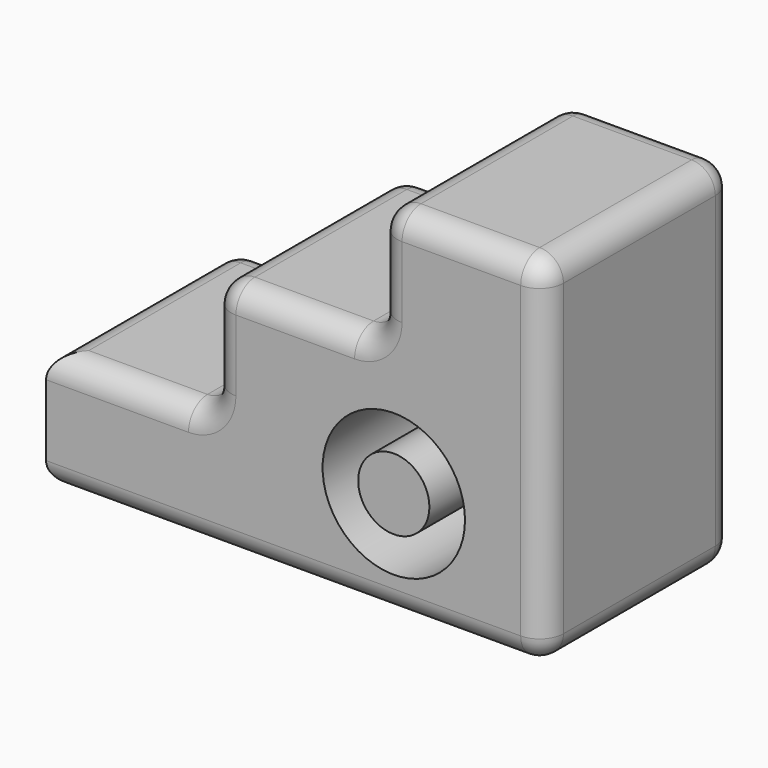
from build123d import *

# Parameters (mm, degrees)
F1_DEPTH      = 50
F2_R          = 15
F2_R_2        = 7.5
F3_DEPTH      = 50
F4_T3_DEPTH   = 50
F4_T6_DEPTH   = 50
F4_S9_W       = 5.1
F4_S9_H       = 5.1
F4_T10_DEPTH  = 5.1
F4_S14_W      = 5.1
F4_S14_H      = 5.1
F4_T15_DEPTH  = 5.1
F4_S19_W      = 5.1
F4_S19_H      = 5.1
F4_T20_DEPTH  = 5.1
F4_S24_W      = 5.1
F4_S24_H      = 5.1
F4_T25_DEPTH  = 5.1
F4_S29_W      = 5.1
F4_S29_H      = 5.1
F4_T30_DEPTH  = 5.1
F4_S34_W      = 5.1
F4_S34_H      = 5.1
F4_T35_DEPTH  = 5.1
F4_S39_W      = 5.1
F4_S39_H      = 5.1
F4_T40_DEPTH  = 5.1
F4_S44_W      = 5.1
F4_S44_H      = 5.1
F4_T45_DEPTH  = 5.1
F4_S49_W      = 5.1
F4_S49_H      = 5.1
F4_T50_DEPTH  = 5.1
F4_S54_W      = 5.1
F4_S54_H      = 5.1
F4_T55_DEPTH  = 5.1
F4_T60_DEPTH  = 57.5
F4_T63_DEPTH  = 40
F4_T66_DEPTH  = 40
F4_T69_DEPTH  = 40
F4_T72_DEPTH  = 25
F4_T75_DEPTH  = 25
F4_T78_DEPTH  = 25
F4_T81_DEPTH  = 42.5
F4_T84_DEPTH  = 25
F4_T87_DEPTH  = 25
F4_T93_DEPTH  = 112.5
F4_T96_DEPTH  = 57.5
F4_T99_DEPTH  = 40
F4_T102_DEPTH = 95
F4_T105_DEPTH = 65
F4_T108_DEPTH = 15
F4_T111_DEPTH = 65
F4_T114_DEPTH = 15
F4_T117_DEPTH = 15
F4_T120_DEPTH = 15
F4_T123_DEPTH = 15
F4_T126_ANGLE = 90
F4_T129_ANGLE = 90
F4_T132_ANGLE = 90
F4_T135_ANGLE = 90


# Not quite as in the source:
# - a fillet or chamfer that OpenCascade refuses, or shapes differently, is made with other operations: its cross-section is extruded or revolved along the edge and cut away or added


with BuildPart() as f1:
    # F0 (on Front) → F1 (new body)
    with BuildSketch(Plane.XZ):
        Polygon((-66.1900187428, 24.934796177), (-66.1900187428, -0.065203823), (38.8099812572, -0.065203823), (38.8099812572, 74.934796177), (3.8099812572, 74.934796177), (3.8099812572, 49.934796177), (-31.1900187428, 49.934796177), (-31.1900187428, 24.934796177), align=None)
    extrude(amount=F1_DEPTH)

    # F2 (on face) → F3 (cut, through all)
    with BuildSketch(Plane.XZ.offset(50)):
        with Locations((7.0711858571, 22.5817617029)):
            Circle(F2_R)
        with Locations((7.0711858571, 22.5817617029)):
            Circle(F2_R_2, mode=Mode.SUBTRACT)
    extrude(amount=-F3_DEPTH, mode=Mode.SUBTRACT)

    # F4: fillet of radius 5 on 24 edges, made by hand


with BuildPart() as f4_tool1:
    # F4_s2 → F4_t3 (new body)
    with BuildSketch(Plane.XZ):
        with BuildLine():
            ThreePointArc((-36.1900187428, 24.934796177), (-32.6544848368, 26.3992622711), (-31.1900187428, 29.934796177))
            Line((-31.1900187428, 29.934796177), (-31.1900187428, 24.934796177))
            Line((-31.1900187428, 24.934796177), (-36.1900187428, 24.934796177))
        make_face()
    extrude(amount=F4_T3_DEPTH)


with BuildPart() as f4_tool4:
    # F4_s5 → F4_t6 (new body)
    with BuildSketch(Plane.XZ):
        with BuildLine():
            ThreePointArc((3.8099812572, 54.934796177), (2.3455151632, 51.3992622711), (-1.1900187428, 49.934796177))
            Line((-1.1900187428, 49.934796177), (3.8099812572, 49.934796177))
            Line((3.8099812572, 49.934796177), (3.8099812572, 54.934796177))
        make_face()
    extrude(amount=F4_T6_DEPTH)


with BuildPart() as f1_1:
    add(f1.part)

    # F4_t7: union F4_tool1, F4_tool4
    add([f4_tool1.part, f4_tool4.part])


with BuildPart() as f4_tool8:
    # F4_s9 → F4_t10 (new body)
    with BuildSketch(Plane.YZ.offset(-61.1900187428)):
        with Locations((-2.45, 22.484796177)):
            Rectangle(F4_S9_W, F4_S9_H)
    extrude(amount=-F4_T10_DEPTH)

    # F4_s11 → F4_t12 (revolve, cut)
    with BuildSketch(Plane(origin=(-61.1900187428, -5, 19.934796177), x_dir=(0, -0.7071067812, -0.7071067812), z_dir=(0, 0.7071067812, -0.7071067812))):
        with BuildLine():
            ThreePointArc((0, -5), (5, 0), (0, 5))
            Line((0, 5), (0, -5))
        make_face()
    revolve(axis=Axis((-61.1900187428, -5, 19.934796177), (-1, 0, 0)), mode=Mode.SUBTRACT)


with BuildPart() as f4_tool13:
    # F4_s14 → F4_t15 (new body)
    with BuildSketch(Plane.XY.offset(44.934796177)):
        with Locations((-28.7400187428, -2.45)):
            Rectangle(F4_S14_W, F4_S14_H)
    extrude(amount=F4_T15_DEPTH)

    # F4_s16 → F4_t17 (revolve, cut)
    with BuildSketch(Plane(origin=(-26.1900187428, -5, 44.934796177), x_dir=(0.7071067812, -0.7071067812, 0), z_dir=(-0.7071067812, -0.7071067812, 0))):
        with BuildLine():
            ThreePointArc((0, -5), (5, 0), (0, 5))
            Line((0, 5), (0, -5))
        make_face()
    revolve(axis=Axis((-26.1900187428, -5, 44.934796177), (0, 0, 1)), mode=Mode.SUBTRACT)


with BuildPart() as f4_tool18:
    # F4_s19 → F4_t20 (new body)
    with BuildSketch(Plane.XY.offset(44.934796177)):
        with Locations((-28.7400187428, -47.55)):
            Rectangle(F4_S19_W, F4_S19_H)
    extrude(amount=F4_T20_DEPTH)

    # F4_s21 → F4_t22 (revolve, cut)
    with BuildSketch(Plane(origin=(-26.1900187428, -45, 44.934796177), x_dir=(0.7071067812, 0.7071067812, 0), z_dir=(0.7071067812, -0.7071067812, 0))):
        with BuildLine():
            ThreePointArc((0, -5), (5, 0), (0, 5))
            Line((0, 5), (0, -5))
        make_face()
    revolve(axis=Axis((-26.1900187428, -45, 44.934796177), (0, 0, 1)), mode=Mode.SUBTRACT)


with BuildPart() as f4_tool23:
    # F4_s24 → F4_t25 (new body)
    with BuildSketch(Plane.YZ.offset(8.8099812572)):
        with Locations((-2.45, 72.484796177)):
            Rectangle(F4_S24_W, F4_S24_H)
    extrude(amount=-F4_T25_DEPTH)

    # F4_s26 → F4_t27 (revolve, cut)
    with BuildSketch(Plane(origin=(8.8099812572, -5, 69.934796177), x_dir=(0, -0.7071067812, -0.7071067812), z_dir=(0, 0.7071067812, -0.7071067812))):
        with BuildLine():
            ThreePointArc((0, -5), (5, 0), (0, 5))
            Line((0, 5), (0, -5))
        make_face()
    revolve(axis=Axis((8.8099812572, -5, 69.934796177), (-1, 0, 0)), mode=Mode.SUBTRACT)


with BuildPart() as f4_tool28:
    # F4_s29 → F4_t30 (new body)
    with BuildSketch(Plane.YZ.offset(8.8099812572)):
        with Locations((-47.55, 72.484796177)):
            Rectangle(F4_S29_W, F4_S29_H)
    extrude(amount=-F4_T30_DEPTH)

    # F4_s31 → F4_t32 (revolve, cut)
    with BuildSketch(Plane(origin=(8.8099812572, -45, 69.934796177), x_dir=(0, 0.7071067812, -0.7071067812), z_dir=(0, 0.7071067812, 0.7071067812))):
        with BuildLine():
            ThreePointArc((0, -5), (5, 0), (0, 5))
            Line((0, 5), (0, -5))
        make_face()
    revolve(axis=Axis((8.8099812572, -45, 69.934796177), (-1, 0, 0)), mode=Mode.SUBTRACT)


with BuildPart() as f4_tool33:
    # F4_s34 → F4_t35 (new body)
    with BuildSketch(Plane.YZ.offset(33.8099812572)):
        with Locations((-2.45, 72.484796177)):
            Rectangle(F4_S34_W, F4_S34_H)
    extrude(amount=F4_T35_DEPTH)

    # F4_s36 → F4_t37 (revolve, cut)
    with BuildSketch(Plane(origin=(33.8099812572, -5, 69.934796177), x_dir=(0, -0.7071067812, -0.7071067812), z_dir=(0, -0.7071067812, 0.7071067812))):
        with BuildLine():
            ThreePointArc((0, -5), (5, 0), (0, 5))
            Line((0, 5), (0, -5))
        make_face()
    revolve(axis=Axis((33.8099812572, -5, 69.934796177), (1, 0, 0)), mode=Mode.SUBTRACT)


with BuildPart() as f4_tool38:
    # F4_s39 → F4_t40 (new body)
    with BuildSketch(Plane.YZ.offset(33.8099812572)):
        with Locations((-47.55, 72.484796177)):
            Rectangle(F4_S39_W, F4_S39_H)
    extrude(amount=F4_T40_DEPTH)

    # F4_s41 → F4_t42 (revolve, cut)
    with BuildSketch(Plane(origin=(33.8099812572, -45, 69.934796177), x_dir=(0, 0.7071067812, -0.7071067812), z_dir=(0, -0.7071067812, -0.7071067812))):
        with BuildLine():
            ThreePointArc((0, -5), (5, 0), (0, 5))
            Line((0, 5), (0, -5))
        make_face()
    revolve(axis=Axis((33.8099812572, -45, 69.934796177), (1, 0, 0)), mode=Mode.SUBTRACT)


with BuildPart() as f4_tool43:
    # F4_s44 → F4_t45 (new body)
    with BuildSketch(Plane.XY.offset(4.934796177)):
        with Locations((36.3599812572, -47.55)):
            Rectangle(F4_S44_W, F4_S44_H)
    extrude(amount=-F4_T45_DEPTH)

    # F4_s46 → F4_t47 (revolve, cut)
    with BuildSketch(Plane(origin=(33.8099812572, -45, 4.934796177), x_dir=(-0.7071067812, 0.7071067812, 0), z_dir=(-0.7071067812, -0.7071067812, 0))):
        with BuildLine():
            ThreePointArc((0, -5), (5, 0), (0, 5))
            Line((0, 5), (0, -5))
        make_face()
    revolve(axis=Axis((33.8099812572, -45, 4.934796177), (0, 0, -1)), mode=Mode.SUBTRACT)


with BuildPart() as f4_tool48:
    # F4_s49 → F4_t50 (new body)
    with BuildSketch(Plane.XY.offset(4.934796177)):
        with Locations((-63.7400187428, -2.45)):
            Rectangle(F4_S49_W, F4_S49_H)
    extrude(amount=-F4_T50_DEPTH)

    # F4_s51 → F4_t52 (revolve, cut)
    with BuildSketch(Plane(origin=(-61.1900187428, -5, 4.934796177), x_dir=(0.7071067812, -0.7071067812, 0), z_dir=(0.7071067812, 0.7071067812, 0))):
        with BuildLine():
            ThreePointArc((0, -5), (5, 0), (0, 5))
            Line((0, 5), (0, -5))
        make_face()
    revolve(axis=Axis((-61.1900187428, -5, 4.934796177), (0, 0, -1)), mode=Mode.SUBTRACT)


with BuildPart() as f4_tool53:
    # F4_s54 → F4_t55 (new body)
    with BuildSketch(Plane.XY.offset(4.934796177)):
        with Locations((36.3599812572, -2.45)):
            Rectangle(F4_S54_W, F4_S54_H)
    extrude(amount=-F4_T55_DEPTH)

    # F4_s56 → F4_t57 (revolve, cut)
    with BuildSketch(Plane(origin=(33.8099812572, -5, 4.934796177), x_dir=(-0.7071067812, -0.7071067812, 0), z_dir=(0.7071067812, -0.7071067812, 0))):
        with BuildLine():
            ThreePointArc((0, -5), (5, 0), (0, 5))
            Line((0, 5), (0, -5))
        make_face()
    revolve(axis=Axis((33.8099812572, -5, 4.934796177), (0, 0, -1)), mode=Mode.SUBTRACT)


with BuildPart() as f4_tool58:
    # F4_s59 → F4_t60 (new body)
    with BuildSketch(Plane.XZ.offset(5)):
        with BuildLine():
            ThreePointArc((-66.1900187428, 19.934796177), (-64.7255526487, 23.470330083), (-61.1900187428, 24.934796177))
            Line((-61.1900187428, 24.934796177), (-66.1900187428, 24.934796177))
            Line((-66.1900187428, 24.934796177), (-66.1900187428, 19.934796177))
        make_face()
    extrude(amount=F4_T60_DEPTH)


with BuildPart() as f4_tool61:
    # F4_s62 → F4_t63 (new body)
    with BuildSketch(Plane.XZ.offset(5)):
        with BuildLine():
            ThreePointArc((-31.1900187428, 44.934796177), (-29.7255526487, 48.470330083), (-26.1900187428, 49.934796177))
            Line((-26.1900187428, 49.934796177), (-31.1900187428, 49.934796177))
            Line((-31.1900187428, 49.934796177), (-31.1900187428, 44.934796177))
        make_face()
    extrude(amount=F4_T63_DEPTH)


with BuildPart() as f4_tool64:
    # F4_s65 → F4_t66 (new body)
    with BuildSketch(Plane.XZ.offset(5)):
        with BuildLine():
            ThreePointArc((8.8099812572, 74.934796177), (5.2744473513, 73.470330083), (3.8099812572, 69.934796177))
            Line((3.8099812572, 69.934796177), (3.8099812572, 74.934796177))
            Line((3.8099812572, 74.934796177), (8.8099812572, 74.934796177))
        make_face()
    extrude(amount=F4_T66_DEPTH)


with BuildPart() as f4_tool67:
    # F4_s68 → F4_t69 (new body)
    with BuildSketch(Plane.XZ.offset(5)):
        with BuildLine():
            ThreePointArc((38.8099812572, 69.934796177), (37.3455151632, 73.470330083), (33.8099812572, 74.934796177))
            Line((33.8099812572, 74.934796177), (38.8099812572, 74.934796177))
            Line((38.8099812572, 74.934796177), (38.8099812572, 69.934796177))
        make_face()
    extrude(amount=F4_T69_DEPTH)


with BuildPart() as f4_tool70:
    # F4_s71 → F4_t72 (new body)
    with BuildSketch(Plane.YZ.offset(33.8099812572)):
        with BuildLine():
            ThreePointArc((0, 69.934796177), (-1.4644660941, 73.470330083), (-5, 74.934796177))
            Line((-5, 74.934796177), (0, 74.934796177))
            Line((0, 74.934796177), (0, 69.934796177))
        make_face()
    extrude(amount=-F4_T72_DEPTH)


with BuildPart() as f4_tool73:
    # F4_s74 → F4_t75 (new body)
    with BuildSketch(Plane.YZ.offset(33.8099812572)):
        with BuildLine():
            ThreePointArc((-50, 69.934796177), (-48.5355339059, 73.470330083), (-45, 74.934796177))
            Line((-45, 74.934796177), (-50, 74.934796177))
            Line((-50, 74.934796177), (-50, 69.934796177))
        make_face()
    extrude(amount=-F4_T75_DEPTH)


with BuildPart() as f4_tool76:
    # F4_s77 → F4_t78 (new body)
    with BuildSketch(Plane.YZ.offset(-1.1900187428)):
        with BuildLine():
            ThreePointArc((-50, 44.934796177), (-48.5355339059, 48.470330083), (-45, 49.934796177))
            Line((-45, 49.934796177), (-50, 49.934796177))
            Line((-50, 49.934796177), (-50, 44.934796177))
        make_face()
    extrude(amount=-F4_T78_DEPTH)


with BuildPart() as f4_tool79:
    # F4_s80 → F4_t81 (new body)
    with BuildSketch(Plane.YZ.offset(-36.1900187428)):
        with BuildLine():
            ThreePointArc((-50, 19.934796177), (-48.5355339059, 23.470330083), (-45, 24.934796177))
            Line((-45, 24.934796177), (-50, 24.934796177))
            Line((-50, 24.934796177), (-50, 19.934796177))
        make_face()
    extrude(amount=-F4_T81_DEPTH)


with BuildPart() as f4_tool82:
    # F4_s83 → F4_t84 (new body)
    with BuildSketch(Plane.YZ.offset(-1.1900187428)):
        with BuildLine():
            ThreePointArc((0, 44.934796177), (-1.4644660941, 48.470330083), (-5, 49.934796177))
            Line((-5, 49.934796177), (0, 49.934796177))
            Line((0, 49.934796177), (0, 44.934796177))
        make_face()
    extrude(amount=-F4_T84_DEPTH)


with BuildPart() as f4_tool85:
    # F4_s86 → F4_t87 (new body)
    with BuildSketch(Plane.YZ.offset(-36.1900187428)):
        with BuildLine():
            ThreePointArc((0, 19.934796177), (-1.4644660941, 23.470330083), (-5, 24.934796177))
            Line((-5, 24.934796177), (0, 24.934796177))
            Line((0, 24.934796177), (0, 19.934796177))
        make_face()
    extrude(amount=-F4_T87_DEPTH)


with BuildPart() as f4_tool88:
    # F4_s89 → F4_t90 (revolve)
    with BuildSketch(Plane.XY.offset(22.5817617029)):
        with BuildLine():
            ThreePointArc((27.0711858571, 0), (23.5356519511, -1.4644660941), (22.0711858571, -5))
            Line((22.0711858571, -5), (22.0711858571, 0))
            Line((22.0711858571, 0), (27.0711858571, 0))
        make_face()
    revolve(axis=Axis((7.0711858571, 0, 22.5817617029), (0, -1, 0)))


with BuildPart() as f4_tool91:
    # F4_s92 → F4_t93 (new body)
    with BuildSketch(Plane.YZ.offset(-78.6900187428)):
        with BuildLine():
            ThreePointArc((-45, -0.065203823), (-48.5355339059, 1.3992622711), (-50, 4.934796177))
            Line((-50, 4.934796177), (-50, -0.065203823))
            Line((-50, -0.065203823), (-45, -0.065203823))
        make_face()
    extrude(amount=F4_T93_DEPTH)


with BuildPart() as f4_tool94:
    # F4_s95 → F4_t96 (new body)
    with BuildSketch(Plane.XZ.offset(5)):
        with BuildLine():
            ThreePointArc((-61.1900187428, -0.065203823), (-64.7255526487, 1.3992622711), (-66.1900187428, 4.934796177))
            Line((-66.1900187428, 4.934796177), (-66.1900187428, -0.065203823))
            Line((-66.1900187428, -0.065203823), (-61.1900187428, -0.065203823))
        make_face()
    extrude(amount=F4_T96_DEPTH)


with BuildPart() as f4_tool97:
    # F4_s98 → F4_t99 (new body)
    with BuildSketch(Plane.XZ.offset(5)):
        with BuildLine():
            ThreePointArc((33.8099812572, -0.065203823), (37.3455151632, 1.3992622711), (38.8099812572, 4.934796177))
            Line((38.8099812572, 4.934796177), (38.8099812572, -0.065203823))
            Line((38.8099812572, -0.065203823), (33.8099812572, -0.065203823))
        make_face()
    extrude(amount=F4_T99_DEPTH)


with BuildPart() as f4_tool100:
    # F4_s101 → F4_t102 (new body)
    with BuildSketch(Plane.YZ.offset(-61.1900187428)):
        with BuildLine():
            ThreePointArc((-5, -0.065203823), (-1.4644660941, 1.3992622711), (0, 4.934796177))
            Line((0, 4.934796177), (0, -0.065203823))
            Line((0, -0.065203823), (-5, -0.065203823))
        make_face()
    extrude(amount=F4_T102_DEPTH)


with BuildPart() as f4_tool103:
    # F4_s104 → F4_t105 (new body)
    with BuildSketch(Plane.XY.offset(4.934796177)):
        with BuildLine():
            ThreePointArc((38.8099812572, -5), (37.3455151632, -1.4644660941), (33.8099812572, 0))
            Line((33.8099812572, 0), (38.8099812572, 0))
            Line((38.8099812572, 0), (38.8099812572, -5))
        make_face()
    extrude(amount=F4_T105_DEPTH)


with BuildPart() as f4_tool106:
    # F4_s107 → F4_t108 (new body)
    with BuildSketch(Plane.XY.offset(19.934796177)):
        with BuildLine():
            ThreePointArc((-66.1900187428, -5), (-64.7255526487, -1.4644660941), (-61.1900187428, 0))
            Line((-61.1900187428, 0), (-66.1900187428, 0))
            Line((-66.1900187428, 0), (-66.1900187428, -5))
        make_face()
    extrude(amount=-F4_T108_DEPTH)


with BuildPart() as f4_tool109:
    # F4_s110 → F4_t111 (new body)
    with BuildSketch(Plane.XY.offset(4.934796177)):
        with BuildLine():
            ThreePointArc((38.8099812572, -45), (37.3455151632, -48.5355339059), (33.8099812572, -50))
            Line((33.8099812572, -50), (38.8099812572, -50))
            Line((38.8099812572, -50), (38.8099812572, -45))
        make_face()
    extrude(amount=F4_T111_DEPTH)


with BuildPart() as f4_tool112:
    # F4_s113 → F4_t114 (new body)
    with BuildSketch(Plane.XY.offset(44.934796177)):
        with BuildLine():
            ThreePointArc((-26.1900187428, 0), (-29.7255526487, -1.4644660941), (-31.1900187428, -5))
            Line((-31.1900187428, -5), (-31.1900187428, 0))
            Line((-31.1900187428, 0), (-26.1900187428, 0))
        make_face()
    extrude(amount=-F4_T114_DEPTH)


with BuildPart() as f4_tool115:
    # F4_s116 → F4_t117 (new body)
    with BuildSketch(Plane.XY.offset(69.934796177)):
        with BuildLine():
            ThreePointArc((8.8099812572, 0), (5.2744473513, -1.4644660941), (3.8099812572, -5))
            Line((3.8099812572, -5), (3.8099812572, 0))
            Line((3.8099812572, 0), (8.8099812572, 0))
        make_face()
    extrude(amount=-F4_T117_DEPTH)


with BuildPart() as f4_tool118:
    # F4_s119 → F4_t120 (new body)
    with BuildSketch(Plane.XY.offset(44.934796177)):
        with BuildLine():
            ThreePointArc((-26.1900187428, -50), (-29.7255526487, -48.5355339059), (-31.1900187428, -45))
            Line((-31.1900187428, -45), (-31.1900187428, -50))
            Line((-31.1900187428, -50), (-26.1900187428, -50))
        make_face()
    extrude(amount=-F4_T120_DEPTH)


with BuildPart() as f4_tool121:
    # F4_s122 → F4_t123 (new body)
    with BuildSketch(Plane.XY.offset(69.934796177)):
        with BuildLine():
            ThreePointArc((8.8099812572, -50), (5.2744473513, -48.5355339059), (3.8099812572, -45))
            Line((3.8099812572, -45), (3.8099812572, -50))
            Line((3.8099812572, -50), (8.8099812572, -50))
        make_face()
    extrude(amount=-F4_T123_DEPTH)


with BuildPart() as f4_tool124:
    # F4_s125 → F4_t126 (revolve)
    with BuildSketch(Plane.XY.offset(54.934796177)):
        with BuildLine():
            ThreePointArc((8.8099812572, -50), (5.2744473513, -48.5355339059), (3.8099812572, -45))
            Line((3.8099812572, -45), (3.8099812572, -50))
            Line((3.8099812572, -50), (8.8099812572, -50))
        make_face()
    revolve(axis=Axis((-1.1900187428, -50, 54.934796177), (0, 1, 0)), revolution_arc=F4_T126_ANGLE)


with BuildPart() as f4_tool127:
    # F4_s128 → F4_t129 (revolve)
    with BuildSketch(Plane.YZ.offset(-36.1900187428)):
        with BuildLine():
            ThreePointArc((-50, 19.934796177), (-48.5355339059, 23.470330083), (-45, 24.934796177))
            Line((-45, 24.934796177), (-50, 24.934796177))
            Line((-50, 24.934796177), (-50, 19.934796177))
        make_face()
    revolve(axis=Axis((-36.1900187428, -50, 29.934796177), (0, -1, 0)), revolution_arc=F4_T129_ANGLE)


with BuildPart() as f4_tool130:
    # F4_s131 → F4_t132 (revolve)
    with BuildSketch(Plane.XY.offset(54.934796177)):
        with BuildLine():
            ThreePointArc((8.8099812572, 0), (5.2744473513, -1.4644660941), (3.8099812572, -5))
            Line((3.8099812572, -5), (3.8099812572, 0))
            Line((3.8099812572, 0), (8.8099812572, 0))
        make_face()
    revolve(axis=Axis((-1.1900187428, 0, 54.934796177), (0, 1, 0)), revolution_arc=F4_T132_ANGLE)


with BuildPart() as f4_tool133:
    # F4_s134 → F4_t135 (revolve)
    with BuildSketch(Plane.YZ.offset(-36.1900187428)):
        with BuildLine():
            ThreePointArc((0, 19.934796177), (-1.4644660941, 23.470330083), (-5, 24.934796177))
            Line((-5, 24.934796177), (0, 24.934796177))
            Line((0, 24.934796177), (0, 19.934796177))
        make_face()
    revolve(axis=Axis((-36.1900187428, 0, 29.934796177), (0, -1, 0)), revolution_arc=F4_T135_ANGLE)


with BuildPart() as f1_2:
    add(f1_1.part)

    # F4_t136: cut F4_tool8, F4_tool13, F4_tool18, F4_tool23, F4_tool28, F4_tool33, F4_tool38, F4_tool43, F4_tool48, F4_tool53, F4_tool58, F4_tool61, F4_tool64, F4_tool67, F4_tool70, F4_tool73, F4_tool76, F4_tool79, F4_tool82, F4_tool85, F4_tool88, F4_tool91, F4_tool94, F4_tool97, F4_tool100, F4_tool103, F4_tool106, F4_tool109, F4_tool112, F4_tool115, F4_tool118, F4_tool121, F4_tool124, F4_tool127, F4_tool130, F4_tool133
    add([f4_tool8.part, f4_tool13.part, f4_tool18.part, f4_tool23.part, f4_tool28.part, f4_tool33.part, f4_tool38.part, f4_tool43.part, f4_tool48.part, f4_tool53.part, f4_tool58.part, f4_tool61.part, f4_tool64.part, f4_tool67.part, f4_tool70.part, f4_tool73.part, f4_tool76.part, f4_tool79.part, f4_tool82.part, f4_tool85.part, f4_tool88.part, f4_tool91.part, f4_tool94.part, f4_tool97.part, f4_tool100.part, f4_tool103.part, f4_tool106.part, f4_tool109.part, f4_tool112.part, f4_tool115.part, f4_tool118.part, f4_tool121.part, f4_tool124.part, f4_tool127.part, f4_tool130.part, f4_tool133.part], mode=Mode.SUBTRACT)

    # F4#s1: fillet of radius 5 on 1 edges, made by hand

    # F4_s1_s1 → F4_s1_t2 (revolve, cut)
    with BuildSketch(Plane.XY.offset(22.5817617029)):
        with BuildLine():
            ThreePointArc((9.5711858571, 0), (13.106719763, -1.4644660941), (14.5711858571, -5))
            Line((14.5711858571, -5), (14.5711858571, 0))
            Line((14.5711858571, 0), (9.5711858571, 0))
        make_face()
    revolve(axis=Axis((7.0711858571, 0, 22.5817617029), (0, -1, 0)), mode=Mode.SUBTRACT)


solid = f1_2.part
